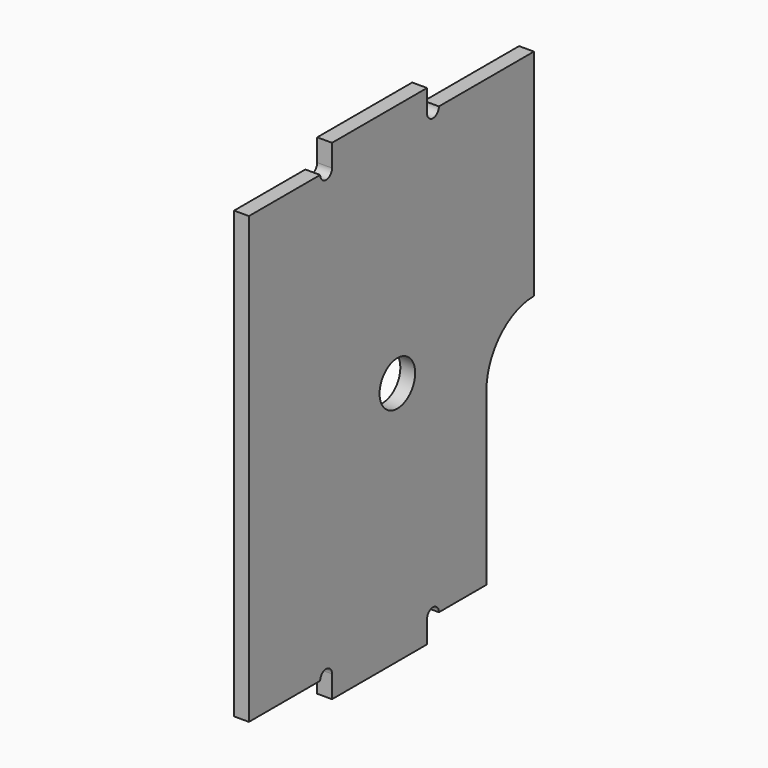
from build123d import *

# Parameters (mm, degrees)
F0_R     = 1.5
F1_DEPTH = 1
F2_R     = 3.99999
F3_R     = 0.5
F4_DEPTH = 25


# Not quite as in the source:
# - a fillet or chamfer is up to 0.001 mm smaller than in the source, because OpenCascade refuses the exact size


with BuildPart() as f1:
    # F0 (on Right) → F1 (new body)
    with BuildSketch(Plane.YZ):
        Polygon((0, 30), (0, 0), (7, 0), (7, -1.5), (15, -1.5), (15, 0), (20, 0), (20, 15.5), (24, 15.5), (24, 30), (15, 30), (15, 31.5), (7, 31.5), (7, 30), align=None)
        with Locations((12.5, 15)):
            Circle(F0_R, mode=Mode.SUBTRACT)
    extrude(amount=F1_DEPTH)

    # F2 (radius 4 in the source; OpenCascade refuses exactly that, so slightly less here)
    f2_edges = [f1.edges().sort_by_distance(p)[0] for p in [
        (0.5, 20, 15.5),
    ]]
    fillet(f2_edges, radius=F2_R)

    # F3 (on face) → F4 (cut)
    with BuildSketch(Plane.YZ.offset(1)):
        with Locations((6.5, 30)):
            Circle(F3_R)
        with Locations((15.5, 30)):
            Circle(F3_R)
        with Locations((6.5, 0)):
            Circle(F3_R)
        with Locations((15.5, 0)):
            Circle(F3_R)
    extrude(amount=-F4_DEPTH, mode=Mode.SUBTRACT)


solid = f1.part
